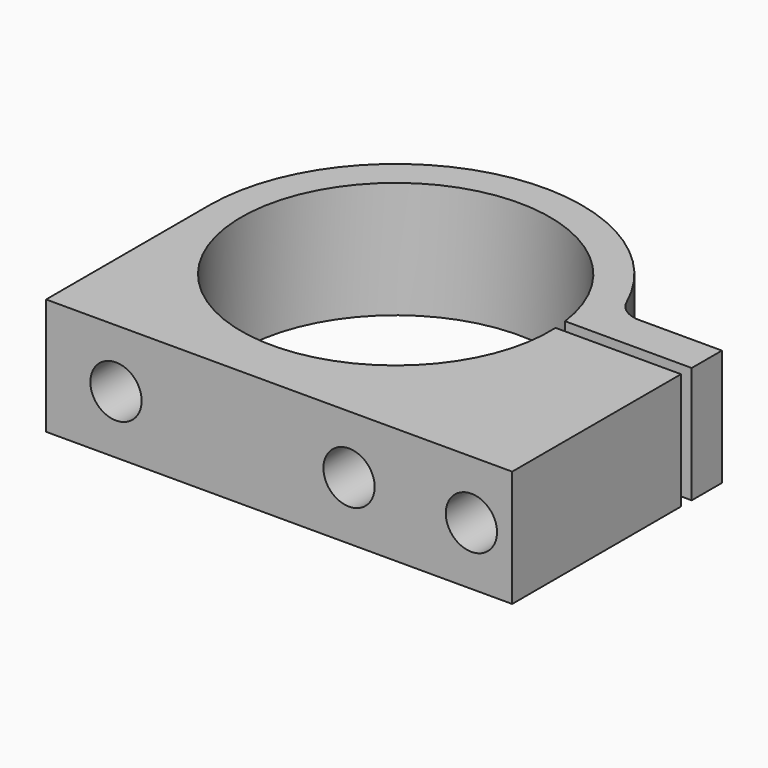
from build123d import *

# Parameters (mm, degrees)
F1_DEPTH  = 20
F2_R      = 26.5
F3_DEPTH  = 20
F4_W      = 50
F4_H      = 2.3
F5_DEPTH  = 20.001
F7_D      = 8.8
F7_DEPTH  = 12
F7_TIP    = 2.6437867237
F8_R      = 5
F10_D     = 8.8
F10_DEPTH = 36.2202316189
F11_D     = 9
F11_DEPTH = 30.7817683811


# Not quite as in the source:
# - a feature of the source that left no trace in its solid (it failed there, or was rolled back) is left out


with BuildPart() as f1:
    # F0 (on Top) → F1 (new body)
    with BuildSketch(Plane.XY):
        with BuildLine():
            ThreePointArc((30.3973683071, 27.5), (-5.0638036184, 49.0968019412), (-32, 17.5))
            Line((-32, 17.5), (-32, -17.5))
            Line((-32, -17.5), (48, -17.5))
            Line((48, -17.5), (48, 27.5))
            Line((48, 27.5), (30.3973683071, 27.5))
        make_face()
    extrude(amount=F1_DEPTH)

    # F2 (on face) → F3 (cut, through all)
    with BuildSketch(Plane.XY.offset(20)):
        with Locations((0, 17.5)):
            Circle(F2_R)
    extrude(amount=-F3_DEPTH, mode=Mode.SUBTRACT)

    # F4 (on face) → F5 (cut, through all)
    with BuildSketch(Plane.XY.offset(20)):
        with Locations((45, 19.8692316189)):
            Rectangle(F4_W, F4_H)
    extrude(amount=-F5_DEPTH, mode=Mode.SUBTRACT)

    # F7
    with Locations(Plane.XZ.offset(17.5)):
        with Locations((-20, 10), (20, 10)):
            Hole(F7_D / 2, depth=F7_DEPTH)
            with Locations((0, 0, -(F7_DEPTH + F7_TIP / 2))):  # 118° drill point
                Cone(0, F7_D / 2, F7_TIP, mode=Mode.SUBTRACT)

    # F8
    f8_edges = [f1.edges().sort_by_distance(p)[0] for p in [
        (30.397368, 27.5, 10),
    ]]
    fillet(f8_edges, radius=F8_R)

    # F10 (through all, one way)
    with BuildSketch(Plane(origin=(0, 18.7192316189, 0), x_dir=(-1, 0, 0), z_dir=(0, 1, 0))):
        with Locations((-41, 10)):
            Circle(F10_D / 2)
    extrude(amount=-F10_DEPTH, mode=Mode.SUBTRACT)

    # F11 (through all, one way)
    with BuildSketch(Plane(origin=(0, 18.7192316189, 0), x_dir=(-1, 0, 0), z_dir=(0, -1, 0))):
        with Locations((-41, -10)):
            Circle(F11_D / 2)
    extrude(amount=-F11_DEPTH, mode=Mode.SUBTRACT)


solid = f1.part
